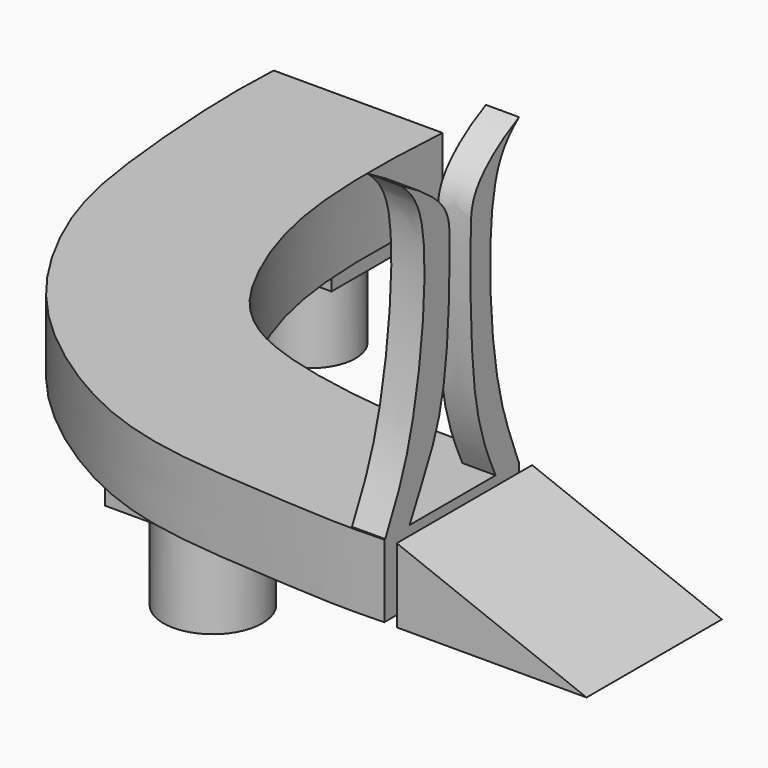
from build123d import *

# Parameters (mm, degrees)
F0_W      = 19.8521018028
F0_H      = 17.1450003982
F1_DEPTH  = 4.318
F0_W_2    = 20.7544714212
F0_H_2    = 17.746578902
F2_R      = 7.0155570226
F3_DEPTH  = 18.542
F4_R      = 7.9467646893
F5_DEPTH  = 18.542
F7_DEPTH  = 11.684
F9_DEPTH  = 5.334
F11_DEPTH = 27.178


# Not quite as in the source:
# - a feature names something its author has since deleted; it is built from what else it names


with BuildPart() as f1:
    # F0 (on Top) → F1 (new body)
    with BuildSketch(Plane.XY):
        with Locations((-76.4005258679, 53.9917089045)):
            Rectangle(F0_W, F0_H)
    extrude(amount=-F1_DEPTH)

    # F2 (on Top) → F3 (join)
    with BuildSketch(Plane.XY):
        with Locations((-76.8517106771, 54.442897439)):
            Circle(F2_R)
    extrude(amount=-F3_DEPTH)



with BuildPart() as f1b:
    # F0 (on Top) → F1, piece 2 (new body)
    with BuildSketch(Plane.XY):
        with Locations((-41.960131377, -8.873289451)):
            Rectangle(F0_W_2, F0_H_2)
    extrude(amount=-F1_DEPTH)

    # F4 (on Top) → F5 (join)
    with BuildSketch(Plane.XY):
        with Locations((-41.960131377, -9.023684077)):
            Circle(F4_R)
    extrude(amount=-F5_DEPTH)


with BuildPart() as f1_1:
    add(f1.part)

    add(f1b.part)  # F7 merges F1b
    # F6 (on Top) → F7 (join)
    with BuildSketch(Plane.XY):
        with BuildLine():
            Line((-63.3161887527, 63.7673661113), (-90.4240001332, 63.7673661113))
            add(Edge.make_bspline(
                [(-90.4240001332, 63.7673661113), (-90.946889777, 54.9811213625), (-89.7279496558, 36.9041024903), (-87.016072715, 18.3355513143), (-76.691665346, -0.8600546564), (-62.441709707, -14.1630605577), (-42.9008739567, -25.1598232125), (-18.8968795163, -26.3894935088), (-8.1307288286, -27.3928058719), (0, -27.0710531622)],
                knots=[0, 0, 0, 0, 0.1597346938, 0.2941128272, 0.434918622, 0.5709144334, 0.7158725886, 0.8630406795, 1, 1, 1, 1], degree=3))
            Line((0, -27.0710531622), (0, 0))
            add(Edge.make_bspline(
                [(-63.3161887527, 63.7673661113), (-63.89678398, 55.0074521155), (-64.5294580411, 37.0316782662), (-57.7315789572, 17.9388743499), (-46.9451503691, 3.0561166092), (-12.5663186528, -0.6113698403), (-4.3614469469, 0), (0, 0)],
                knots=[0, 0, 0, 0, 0.224429372, 0.4162435973, 0.596206914, 0.8431707494, 1, 1, 1, 1], degree=3))
        make_face()
    extrude(amount=F7_DEPTH)

    # F8 (on Right) → F9 (join)
    with BuildSketch(Plane.YZ):
        with BuildLine():
            add(Edge.make_bspline(
                [(-27.004128322, 11.4234443754), (-24.9170712549, 15.6206381214), (-20.4925139948, 24.3371562752), (-17.3602385126, 54.0539118613), (-22.0986272096, 58.9304288492), (-23.8349272719, 60.4167338461)],
                knots=[0, 0, 0, 0, 0.323201421, 0.7663718509, 1, 1, 1, 1], degree=3))
            Line((-27.004128322, 11.4234443754), (-22.0986272096, 11.4234443754))
            add(Edge.make_bspline(
                [(-23.8349272719, 60.4167338461), (-20.3755259414, 58.5333244768), (-13.8305290902, 54.1752420005), (-13.9828351318, 46.9464555143), (-14.1446804387, 24.1753330063), (-19.9336931034, 16.1872758203), (-22.0986272096, 11.4234443754)],
                knots=[0, 0, 0, 0, 0.2285560301, 0.4078773473, 0.7293386816, 1, 1, 1, 1], degree=3))
        make_face()
        with BuildLine():
            Line((-4.5958016999, 11.4234443754), (0, 11.4234443754))
            add(Edge.make_bspline(
                [(0, 11.4234443754), (-1.5558292644, 15.6668477759), (-5.6052633039, 24.4549985378), (-6.7930231719, 54.1771953118), (-1.846077584, 58.9573064034), (0, 60.4167338461)],
                knots=[0, 0, 0, 0, 0.3197343851, 0.7628518919, 1, 1, 1, 1], degree=3))
            add(Edge.make_bspline(
                [(0, 60.4167338461), (-3.8426967978, 58.6067863753), (-9.5985845649, 54.1181159991), (-9.7955748005, 46.9674516518), (-9.7992443925, 24.4412973301), (-6.835249773, 16.1643384386), (-4.5958016999, 11.4234443754)],
                knots=[0, 0, 0, 0, 0.2287475428, 0.4096869795, 0.733305586, 1, 1, 1, 1], degree=3))
        make_face()
    extrude(amount=-F9_DEPTH)


with BuildPart() as f11:
    # F10 (on Front) → F11 (new body)
    with BuildSketch(Plane.XZ):
        Polygon((32.5760170817, 0), (2.0960178226, 11.903770268), (2.0960178226, 0), align=None)
    extrude(amount=F11_DEPTH)


solid = Compound([f1_1.part, f11.part])
